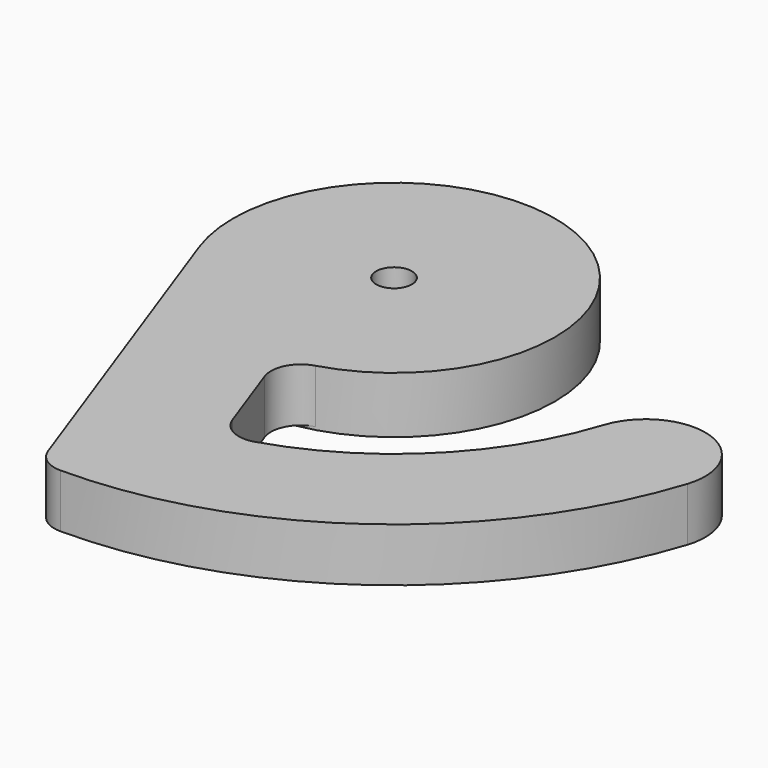
from build123d import *

# Parameters (mm, degrees)
F1_DEPTH  = 6
F2_R      = 3
F3_DEPTH  = 2
F4_R      = 2.5
F5_DEPTH  = 25
F6_DEPTH  = 1.5
F7_R      = 6.9999998683
F8_DEPTH  = 2
F9_DEPTH  = 25
F10_R     = 10
F10_R_2   = 2.5
F11_DEPTH = 2
F12_DEPTH = 1.6
F13_R     = 27
F13_R_2   = 2.5
F14_DEPTH = 1.5
F15_R     = 27
F15_R_2   = 26
F16_DEPTH = 8
F17_R     = 26
F17_R_2   = 25
F18_DEPTH = 1
F19_R     = 3
F20_DEPTH = 5
F21_R     = 10
F21_R_2   = 9.5
F22_DEPTH = 2.1
F24_DEPTH = 9
F25_R     = 5


with BuildPart() as f1:
    # F0 (on Top) → F1 (new body)
    with BuildSketch(Plane.XY):
        Polygon((4.71808, -0.549743), (4.75, 0), (4.71808, 0.549743), (5.165056, 0.601824), (5.611973, 0.654414), (6.042571, 0.835065), (6.451897, 1.12939), (6.835156, 1.510179), (6.761481, 1.811733), (6.674508, 2.109724), (6.152202, 2.247869), (5.650552, 2.298099), (5.187318, 2.239248), (4.773982, 2.061333), (4.360849, 1.882949), (4.113621, 2.375), (3.811106, 2.835132), (4.172158, 3.103723), (4.532904, 3.372726), (4.815488, 3.744473), (5.022812, 4.204029), (5.164329, 4.725432), (4.949747, 4.949747), (4.725432, 5.164329), (4.204029, 5.022812), (3.744473, 4.815488), (3.372726, 4.532904), (3.103723, 4.172158), (2.835132, 3.811106), (2.375, 4.113621), (1.882949, 4.360849), (2.061333, 4.773982), (2.239248, 5.187318), (2.298099, 5.650552), (2.247869, 6.152202), (2.109724, 6.674508), (1.811733, 6.761481), (1.510179, 6.835156), (1.12939, 6.451897), (0.835065, 6.042571), (0.654414, 5.611973), (0.601824, 5.165056), (0.549743, 4.71808), (0, 4.75), (-0.549743, 4.71808), (-0.601824, 5.165056), (-0.654414, 5.611973), (-0.835065, 6.042571), (-1.12939, 6.451897), (-1.510179, 6.835156), (-1.811733, 6.761481), (-2.109724, 6.674508), (-2.247869, 6.152202), (-2.298099, 5.650552), (-2.239248, 5.187318), (-2.061333, 4.773982), (-1.882949, 4.360849), (-2.375, 4.113621), (-2.835132, 3.811106), (-3.103723, 4.172158), (-3.372726, 4.532904), (-3.744473, 4.815488), (-4.204029, 5.022812), (-4.725432, 5.164329), (-4.949747, 4.949747), (-5.164329, 4.725432), (-5.022812, 4.204029), (-4.815488, 3.744473), (-4.532904, 3.372726), (-4.172158, 3.103723), (-3.811106, 2.835132), (-4.113621, 2.375), (-4.360849, 1.882949), (-4.773982, 2.061333), (-5.187318, 2.239248), (-5.650552, 2.298099), (-6.152202, 2.247869), (-6.674508, 2.109724), (-6.761481, 1.811733), (-6.835156, 1.510179), (-6.451897, 1.12939), (-6.042571, 0.835065), (-5.611973, 0.654414), (-5.165056, 0.601824), (-4.71808, 0.549743), (-4.75, 0), (-4.71808, -0.549743), (-5.165056, -0.601824), (-5.611973, -0.654414), (-6.042571, -0.835065), (-6.451897, -1.12939), (-6.835156, -1.510179), (-6.761481, -1.811733), (-6.674508, -2.109724), (-6.152202, -2.247869), (-5.650552, -2.298099), (-5.187318, -2.239248), (-4.773982, -2.061333), (-4.360849, -1.882949), (-4.113621, -2.375), (-3.811106, -2.835132), (-4.172158, -3.103723), (-4.532904, -3.372726), (-4.815488, -3.744473), (-5.022812, -4.204029), (-5.164329, -4.725432), (-4.949747, -4.949747), (-4.725432, -5.164329), (-4.204029, -5.022812), (-3.744473, -4.815488), (-3.372726, -4.532904), (-3.103723, -4.172158), (-2.835132, -3.811106), (-2.375, -4.113621), (-1.882949, -4.360849), (-2.061333, -4.773982), (-2.239248, -5.187318), (-2.298099, -5.650552), (-2.247869, -6.152202), (-2.109724, -6.674508), (-1.811733, -6.761481), (-1.510179, -6.835156), (-1.12939, -6.451897), (-0.835065, -6.042571), (-0.654414, -5.611973), (-0.601824, -5.165056), (-0.549743, -4.71808), (0, -4.75), (0.549743, -4.71808), (0.601824, -5.165056), (0.654414, -5.611973), (0.835065, -6.042571), (1.12939, -6.451897), (1.510179, -6.835156), (1.811733, -6.761481), (2.109724, -6.674508), (2.247869, -6.152202), (2.298099, -5.650552), (2.239248, -5.187318), (2.061333, -4.773982), (1.882949, -4.360849), (2.375, -4.113621), (2.835132, -3.811106), (3.103723, -4.172158), (3.372726, -4.532904), (3.744473, -4.815488), (4.204029, -5.022812), (4.725432, -5.164329), (4.949747, -4.949747), (5.164329, -4.725432), (5.022812, -4.204029), (4.815488, -3.744473), (4.532904, -3.372726), (4.172158, -3.103723), (3.811106, -2.835132), (4.113621, -2.375), (4.360849, -1.882949), (4.773982, -2.061333), (5.187318, -2.239248), (5.650552, -2.298099), (6.152202, -2.247869), (6.674508, -2.109724), (6.761481, -1.811733), (6.835156, -1.510179), (6.451897, -1.12939), (6.042571, -0.835065), (5.611973, -0.654414), (5.165056, -0.601824), align=None)
    extrude(amount=F1_DEPTH)

    # F2 (on face) → F3 (cut)
    with BuildSketch(Plane(origin=(0, 0, 0), x_dir=(1, 0, 0), z_dir=(0, 0, -1))):
        Circle(F2_R)
    extrude(amount=-F3_DEPTH, mode=Mode.SUBTRACT)

    # F4 (on face) → F5 (cut)
    with BuildSketch(Plane.XY.offset(6)):
        Circle(F4_R)
    extrude(amount=-F5_DEPTH, mode=Mode.SUBTRACT)

    # F6 (cut): a face of the model
    f6_faces = [f1.faces().sort_by_distance(p)[0] for p in [
        (4.541037661, -0.2636651096, 6),
    ]]
    extrude(f6_faces, amount=-F6_DEPTH, mode=Mode.SUBTRACT)

    # F7 (on face) → F8 (join)
    with BuildSketch(Plane.XY.offset(4.5)):
        Circle(F7_R)
    extrude(amount=F8_DEPTH)

    # F9 (cut): a face of the model
    f9_faces = [f1.faces().sort_by_distance(p)[0] for p in [
        (0, 0, 4.5),
    ]]
    extrude(f9_faces, amount=-F9_DEPTH, mode=Mode.SUBTRACT)

    # F10 (on face) → F11 (join)
    with BuildSketch(Plane.XY.offset(6.5)):
        Circle(F10_R)
        Circle(F10_R_2, mode=Mode.SUBTRACT)
    extrude(amount=-F11_DEPTH)

    # F12 (add): a face of the model
    f12_faces = [f1.faces().sort_by_distance(p)[0] for p in [
        (-9.7171572875, 0, 6.5),
    ]]
    extrude(f12_faces, amount=F12_DEPTH)

    # F13 (on face) → F14 (join)
    with BuildSketch(Plane.XY.offset(8.1)):
        Circle(F13_R)
        Circle(F13_R_2, mode=Mode.SUBTRACT)
    extrude(amount=-F14_DEPTH)

    # F15 (on face) → F16 (join)
    with BuildSketch(Plane(origin=(0, 0, 6.6), x_dir=(1, 0, 0), z_dir=(0, 0, -1))):
        Circle(F15_R)
        Circle(F15_R_2, mode=Mode.SUBTRACT)
    extrude(amount=F16_DEPTH)

    # F17 (on face) → F18 (join)
    with BuildSketch(Plane(origin=(0, 0, 6.6), x_dir=(1, 0, 0), z_dir=(0, 0, -1))):
        Circle(F17_R)
        Circle(F17_R_2, mode=Mode.SUBTRACT)
    extrude(amount=F18_DEPTH)

    # F19 (on face) → F20 (cut)
    with BuildSketch(Plane.XY.offset(8.1)):
        Circle(F19_R)
    extrude(amount=-F20_DEPTH, mode=Mode.SUBTRACT)

    # F21 (on face) → F22 (cut)
    with BuildSketch(Plane(origin=(0, 0, 4.5), x_dir=(1, 0, 0), z_dir=(0, 0, -1))):
        Circle(F21_R)
        Circle(F21_R_2, mode=Mode.SUBTRACT)
    extrude(amount=-F22_DEPTH, mode=Mode.SUBTRACT)

    # F23 (on face) → F24 (join)
    with BuildSketch(Plane.XY.offset(8.1)):
        with BuildLine():
            ThreePointArc((2.2391355157, -26.906992997), (-14.5983382404, -22.7131794476), (-25.4064661201, -9.1384615385))
            Line((-25.4064661201, -9.1384615385), (-4.7049011333, -66.6923076923))
            ThreePointArc((-4.7049011333, -66.6923076923), (-2.8756270219, -69.0903262988), (0, -70))
            ThreePointArc((0, -70), (41.1449676605, -56.6311896062), (66.5739561407, -21.6311896062))
            Line((66.5739561407, -21.6311896062), (47.5528258148, -15.4508497187))
            ThreePointArc((47.5528258148, -15.4508497187), (33.3706178549, -37.2344177339), (10.1695484735, -48.954880082))
            Line((10.1695484735, -48.954880082), (2.2391355157, -26.906992997))
        make_face()
        with BuildLine():
            ThreePointArc((66.5739561407, -21.6311896062), (60.1535609215, -9.0304544995), (47.5528258148, -15.4508497187))
            Line((47.5528258148, -15.4508497187), (66.5739561407, -21.6311896062))
        make_face()
    extrude(amount=-F24_DEPTH)

    # F25
    f25_edges = [f1.edges().sort_by_distance(p)[0] for p in [
        (10.169548, -48.95488, 3.6),
        (27, 0, 3.35),
        (2.239136, -26.906993, 3.6),
    ]]
    fillet(f25_edges, radius=F25_R)


solid = f1.part
